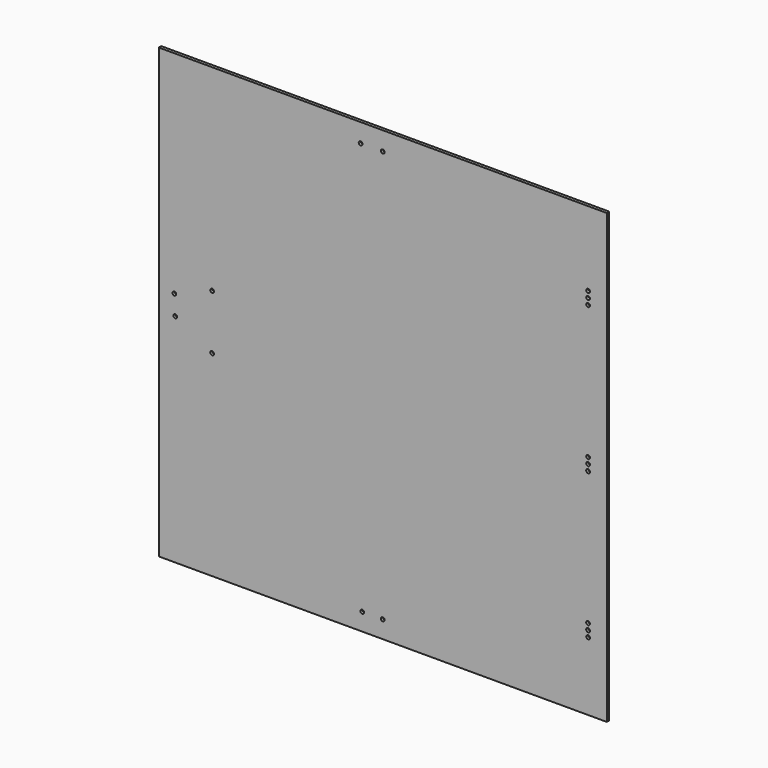
from build123d import *

# Parameters (mm, degrees)
F0_W           = 38.1
F0_H           = 914.4
F0_W_2         = 876.3
F1_DEPTH       = 6.35
F2_D           = 7.62
F2_CSINK_D     = 9.525
F2_CSINK_ANGLE = 90


# Not quite as in the source:
# - a feature names something its author has since deleted; it is built from what else it names


with BuildPart() as f1:
    # F0 (on Front) → F1 (new body)
    with BuildSketch(Plane.XZ):
        with Locations((438.15, 0)):
            Rectangle(F0_W, F0_H)
        with Locations((-19.05, 0)):
            Rectangle(F0_W_2, F0_H)
    extrude(amount=F1_DEPTH)

    # F2 (through all)
    with Locations(Plane(origin=(0, 0, 0), x_dir=(1, 0, 0), z_dir=(0, 1, 0))):
        with Locations((419.1, -304.8), (419.1, -292.1), (419.1, -279.4), (419.1, -6.35), (419.1, 19.05), (419.1, 317.5), (419.1, 304.8), (419.1, 292.1), (419.1, 6.35), (-348.3093082905, -55.6258931756), (-348.3093082905, 56.5741732717), (-423.6675798893, 14.7084780037), (-425.3421723843, -25.482589379), (-45.2016629279, -419.0201461315), (0, -419.0201461315), (-41.8524071574, 421.6430485249), (0, 421.6430485249)):
            CounterSinkHole(F2_D / 2, F2_CSINK_D / 2, counter_sink_angle=F2_CSINK_ANGLE)


solid = f1.part
